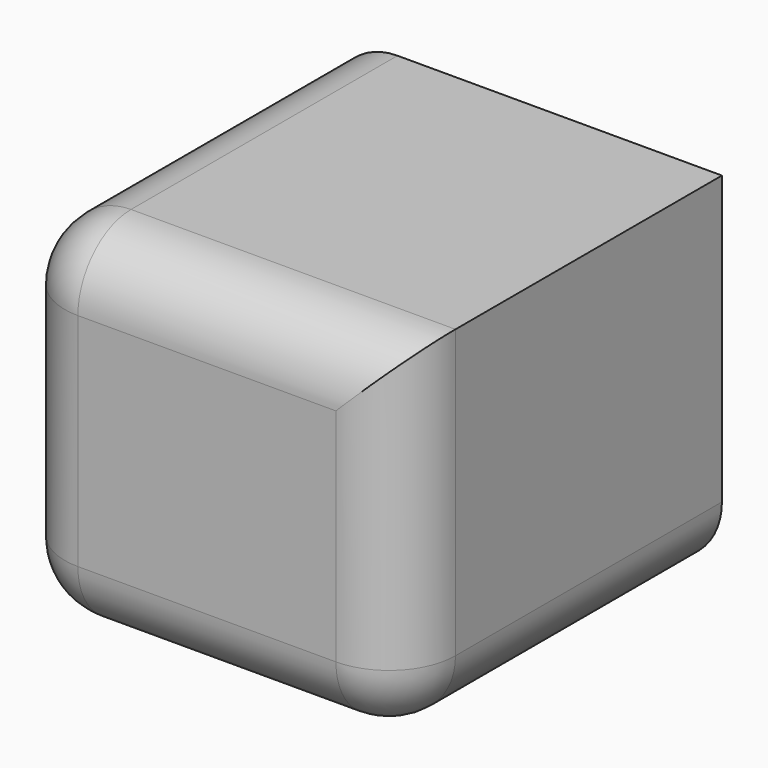
from build123d import *

# Parameters (mm, degrees)
F1_W     = 71.663826704
F1_H     = 64.8628622293
F2_DEPTH = 73.2403695583
F5_R     = 12.1768440653


# Not quite as in the source:
# - the program builds the solid bodies; features that only make, move or delete a surface that nothing else refers to are left out


with BuildPart() as f2:
    # F1 (on face) → F2 (new body)
    with BuildSketch(Plane.XZ):
        with Locations((1.3996511698, -0.3036260605)):
            Rectangle(F1_W, F1_H)
    extrude(amount=F2_DEPTH)

    # F5
    f5_edges = [f2.edges().sort_by_distance(p)[0] for p in [
        (-34.432262, -36.620185, -32.735057),
        (37.231565, -36.620185, -32.735057),
        (-34.432262, -36.620185, 32.127805),
        (-34.432262, -73.24037, -0.303626),
        (1.399651, -73.24037, 32.127805),
        (37.231565, -73.24037, -0.303626),
        (1.399651, -73.24037, -32.735057),
    ]]
    fillet(f5_edges, radius=F5_R)


solid = f2.part
